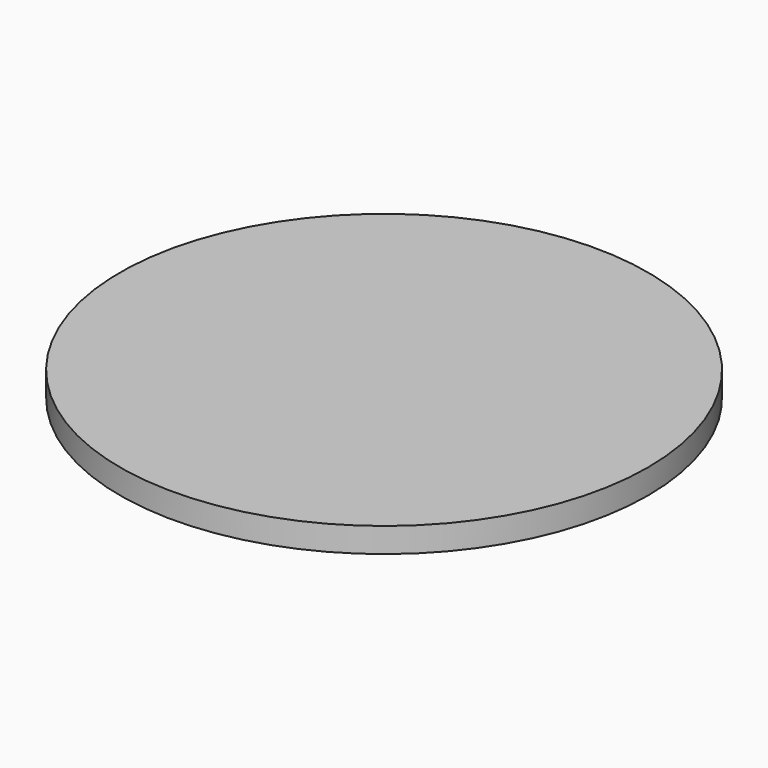
from build123d import *

# Parameters (mm, degrees)
F0_R     = 101.6
F0_R_2   = 98.425
F1_DEPTH = 9.525
F2_R     = 98.425
F3_DEPTH = 3.175


# Not quite as in the source:
# - a length typed as a fraction of an inch, garbled in the dataset ("3 / 203.2 mm" for 3/8 in), is restored


with BuildPart() as f1:
    # F0 (on Top) → F1 (new body)
    with BuildSketch(Plane.XY):
        Circle(F0_R)
        Circle(F0_R_2, mode=Mode.SUBTRACT)
    extrude(amount=-F1_DEPTH)

    # F2 (on Top) → F3 (join)
    with BuildSketch(Plane.XY):
        Circle(F2_R)
    extrude(amount=-F3_DEPTH)


solid = f1.part
